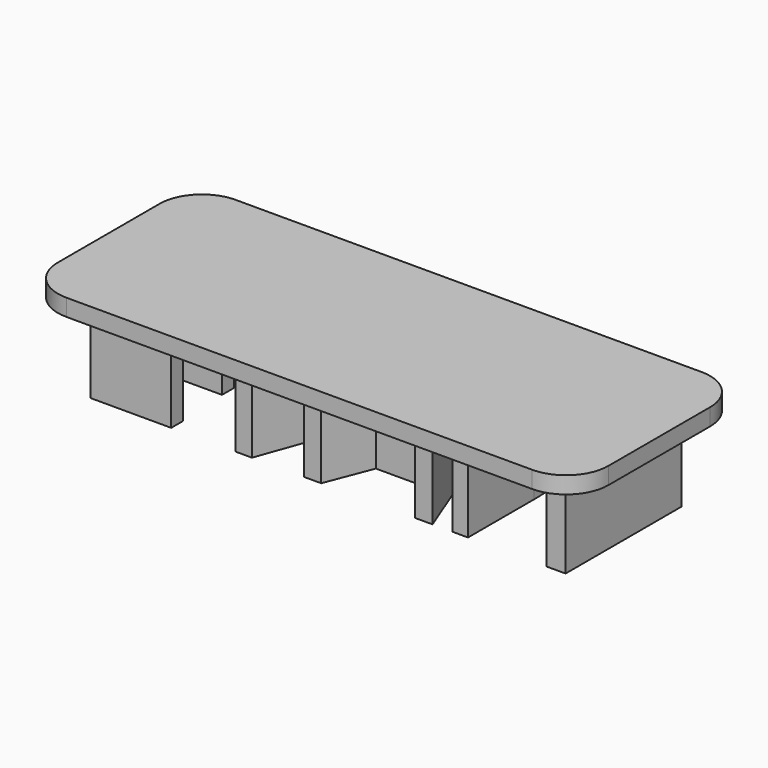
from build123d import *

# Parameters (mm, degrees)
F0_TEXT_SIZE = 30.4229569557
F1_DEPTH     = 12.7
F2_W         = 82.55
F2_H         = 31.75
F3_DEPTH     = 2.54
F4_R         = 6.35


# Not quite as in the source:
# - Text() gives the source's letters only with a copy of the font that has no kerning and outlines rounded to 1/6400 em; it was checked with that copy


with BuildPart() as f1:
    # F0 (on Top) → F1 (new body)
    with BuildSketch(Plane.XY):
        with Locations((-38.1, -11.1252)):
            Text('EVAN', F0_TEXT_SIZE, font='Open Sans', text_align=(TextAlign.LEFT, TextAlign.BOTTOM))
    extrude(amount=-F1_DEPTH)


with BuildPart() as f3:
    # F2 (on Top) → F3 (new body)
    with BuildSketch(Plane.XY):
        Rectangle(F2_W, F2_H)
    extrude(amount=F3_DEPTH)

    # F4
    f4_edges = [f3.edges().sort_by_distance(p)[0] for p in [
        (-41.275, 15.875, 1.27),
        (-41.275, -15.875, 1.27),
        (41.275, -15.875, 1.27),
        (41.275, 15.875, 1.27),
    ]]
    fillet(f4_edges, radius=F4_R)


solid = Compound([f1.part, f3.part])
